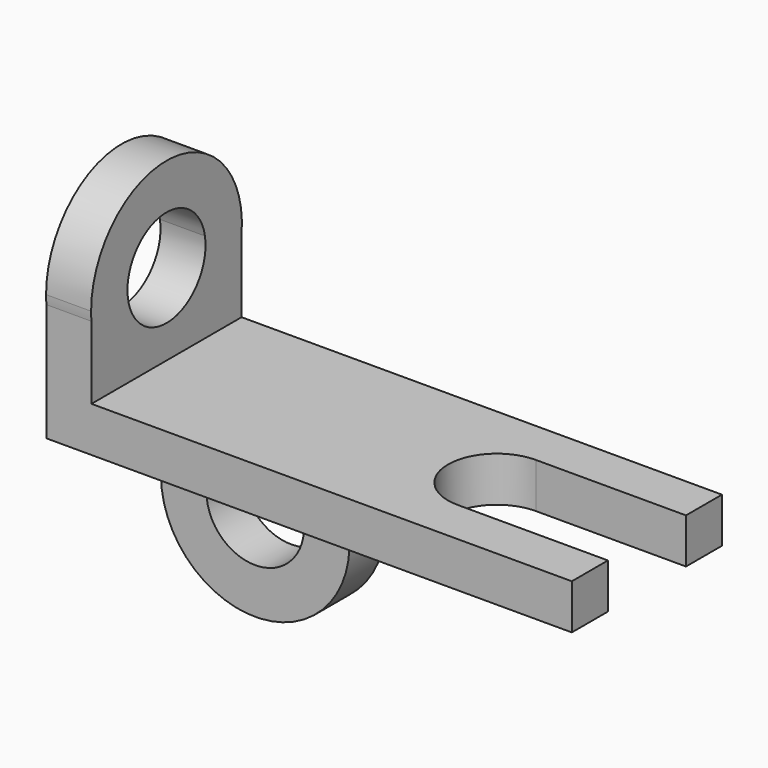
from build123d import *

# Parameters (mm, degrees)
F1_DEPTH = 6
F3_DEPTH = 6
F5_DEPTH = 6


# Not quite as in the source:
# - a feature names something its author has since deleted; it is built from what else it names


with BuildPart() as f1:
    # F0 (on Top) → F1 (new body)
    with BuildSketch(Plane.XY):
        with BuildLine():
            Line((33, 13.8434663415), (-31, 13.8434663415))
            Line((-31, 13.8434663415), (-31, -11.1565336585))
            Line((-31, -11.1565336585), (33, -11.1565336585))
            Line((33, -11.1565336585), (33, -5.1422468387))
            Line((33, -5.1422468387), (13, -5.1422468387))
            ThreePointArc((13, -5.1422468387), (6.5, 1.3577531613), (13, 7.8577531613))
            Line((13, 7.8577531613), (33, 7.8577531613))
            Line((33, 7.8577531613), (33, 13.8434663415))
        make_face()
    extrude(amount=F1_DEPTH)

    # F2 (on face) → F3 (join)
    with BuildSketch(Plane(origin=(-31, 0, 0), x_dir=(0, -1, 0), z_dir=(-1, 0, 0))):
        with BuildLine():
            Line((-13.8434663415, 0), (11.1565336585, 0))
            Line((11.1565336585, 0), (11.1565336585, 15.6810280987))
            ThreePointArc((11.1565336585, 15.6810280987), (-1.3434663415, 4.3280202761), (-13.8434663415, 15.6810280987))
            Line((-13.8434663415, 15.6810280987), (-13.8434663415, 0))
        make_face()
        with BuildLine():
            ThreePointArc((-13.8434663415, 15.6810280987), (-1.3434663415, 4.3280202761), (11.1565336585, 15.6810280987))
            Line((11.1565336585, 15.6810280987), (11.1565336585, 18))
            Line((11.1565336585, 18), (5.0603540757, 18))
            ThreePointArc((5.0603540757, 18), (5.1324441239, 17.4450522775), (5.1565336585, 16.8859604746))
            ThreePointArc((5.1565336585, 16.8859604746), (-1.9025581444, 10.4100500092), (-7.7472867587, 18))
            Line((-7.7472867587, 18), (-13.8434663415, 18))
            Line((-13.8434663415, 18), (-13.8434663415, 15.6810280987))
        make_face()
        with BuildLine():
            Line((11.1565336585, 18), (11.1565336585, 15.6810280987))
            ThreePointArc((11.1565336585, 15.6810280987), (11.1999804438, 16.2827981629), (11.2144738571, 16.8859604746))
            ThreePointArc((11.2144738571, 16.8859604746), (-1.9466286532, 29.4294072599), (-13.8434663415, 15.6810280987))
            Line((-13.8434663415, 15.6810280987), (-13.8434663415, 18))
            Line((-13.8434663415, 18), (-7.7472867587, 18))
            ThreePointArc((-7.7472867587, 18), (-1.3434663415, 23.3859604746), (5.0603540757, 18))
            Line((5.0603540757, 18), (11.1565336585, 18))
        make_face()
    extrude(amount=F3_DEPTH)

    # F4 (on face) → F5 (join)
    with BuildSketch(Plane(origin=(0, 13.8434663415, 0), x_dir=(-1, 0, 0), z_dir=(0, 1, 0))):
        with BuildLine():
            Line((36.8821393698, 6), (11.8821393698, 6))
            Line((11.8821393698, 6), (11.8821393698, -10.7988112149))
            ThreePointArc((11.8821393698, -10.7988112149), (24.3821393698, 0.5575815545), (36.8821393698, -10.7988112149))
            Line((36.8821393698, -10.7988112149), (36.8821393698, 6))
        make_face()
        with BuildLine():
            ThreePointArc((36.8821393698, -10.7988112149), (24.3821393698, 0.5575815545), (11.8821393698, -10.7988112149))
            Line((11.8821393698, -10.7988112149), (11.8821393698, -12))
            Line((11.8821393698, -12), (17.8821393698, -12))
            ThreePointArc((17.8821393698, -12), (24.3821393698, -5.5), (30.8821393698, -12))
            Line((30.8821393698, -12), (36.8821393698, -12))
            Line((36.8821393698, -12), (36.8821393698, -10.7988112149))
        make_face()
        with BuildLine():
            Line((11.8821393698, -12), (11.8821393698, -10.7988112149))
            ThreePointArc((11.8821393698, -10.7988112149), (23.7808552995, -24.5431779053), (36.9397209243, -12))
            ThreePointArc((36.9397209243, -12), (36.9253172752, -11.3987159297), (36.8821393698, -10.7988112149))
            Line((36.8821393698, -10.7988112149), (36.8821393698, -12))
            Line((36.8821393698, -12), (30.8821393698, -12))
            ThreePointArc((30.8821393698, -12), (24.3821393698, -18.5), (17.8821393698, -12))
            Line((17.8821393698, -12), (11.8821393698, -12))
        make_face()
    extrude(amount=-F5_DEPTH)


solid = f1.part
